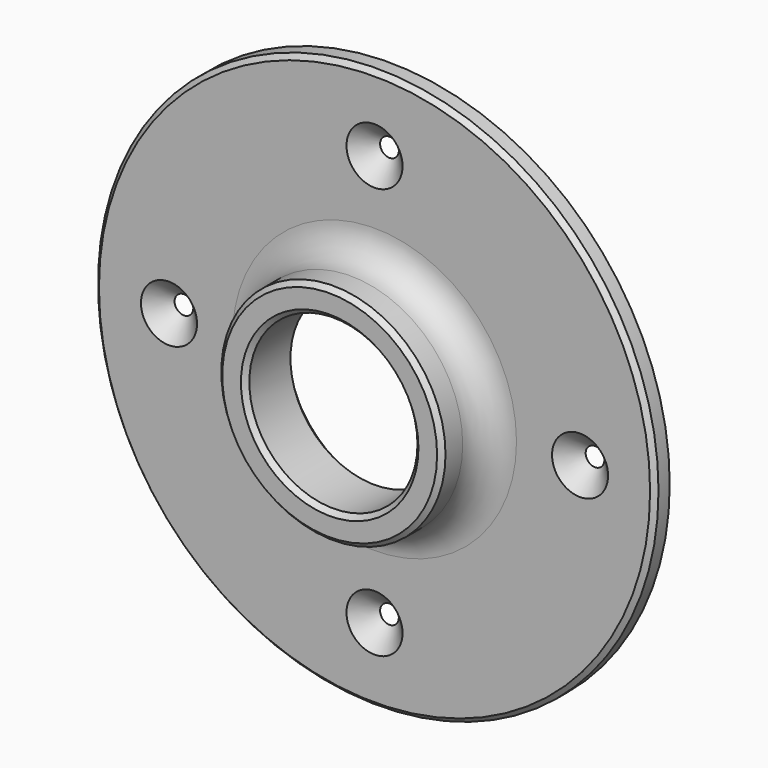
from build123d import *

# Parameters (mm, degrees)
F0_R     = 47.625
F0_R_2   = 1.5875
F0_R_3   = 19.05
F0_R_4   = 14.2875
F1_DEPTH = 3.175
F2_DEPTH = 12.7
F3_SIZE  = 3.17499
F4_SIZE  = 0.79375
F5_SIZE  = 0.79375
F6_R     = 5.08
F7_SIZE  = 3.175


# Not quite as in the source:
# - a fillet or chamfer is up to 0.001 mm smaller than in the source, because OpenCascade refuses the exact size


with BuildPart() as f1:
    # F0 (on Front) → F1 (new body)
    with BuildSketch(Plane.XZ):
        Circle(F0_R)
        with Locations((0, -34.925)):
            Circle(F0_R_2, mode=Mode.SUBTRACT)
        with Locations((-34.925, 0)):
            Circle(F0_R_2, mode=Mode.SUBTRACT)
        Circle(F0_R_3, mode=Mode.SUBTRACT)
        with Locations((34.925, 0)):
            Circle(F0_R_2, mode=Mode.SUBTRACT)
        with Locations((0, 34.925)):
            Circle(F0_R_2, mode=Mode.SUBTRACT)
        Circle(F0_R_3)
        Circle(F0_R_4, mode=Mode.SUBTRACT)
    extrude(amount=F1_DEPTH)

    # F0 (on Front) → F2 (join)
    with BuildSketch(Plane.XZ):
        Circle(F0_R_3)
        Circle(F0_R_4, mode=Mode.SUBTRACT)
    extrude(amount=F2_DEPTH)

    # F3 (size 3.175 in the source; OpenCascade refuses exactly that, so slightly less here)
    f3_edges = [f1.edges().sort_by_distance(p)[0] for p in [
        (-1.5875, -3.175, 34.925),
        (-36.5125, -3.175, 0),
        (33.3375, -3.175, 0),
        (-1.5875, -3.175, -34.925),
    ]]
    chamfer(f3_edges, length=F3_SIZE)

    # F4
    f4_edges = [f1.edges().sort_by_distance(p)[0] for p in [
        (-47.625, -3.175, 0),
    ]]
    chamfer(f4_edges, length=F4_SIZE)

    # F5
    f5_edges = [f1.edges().sort_by_distance(p)[0] for p in [
        (-19.05, -12.7, 0),
        (-14.2875, -12.7, 0),
    ]]
    chamfer(f5_edges, length=F5_SIZE)

    # F6
    f6_edges = [f1.edges().sort_by_distance(p)[0] for p in [
        (-19.05, -3.175, 0),
    ]]
    fillet(f6_edges, radius=F6_R)

    # F7
    f7_edges = [f1.edges().sort_by_distance(p)[0] for p in [
        (-14.2875, 0, 0),
    ]]
    chamfer(f7_edges, length=F7_SIZE)


solid = f1.part
